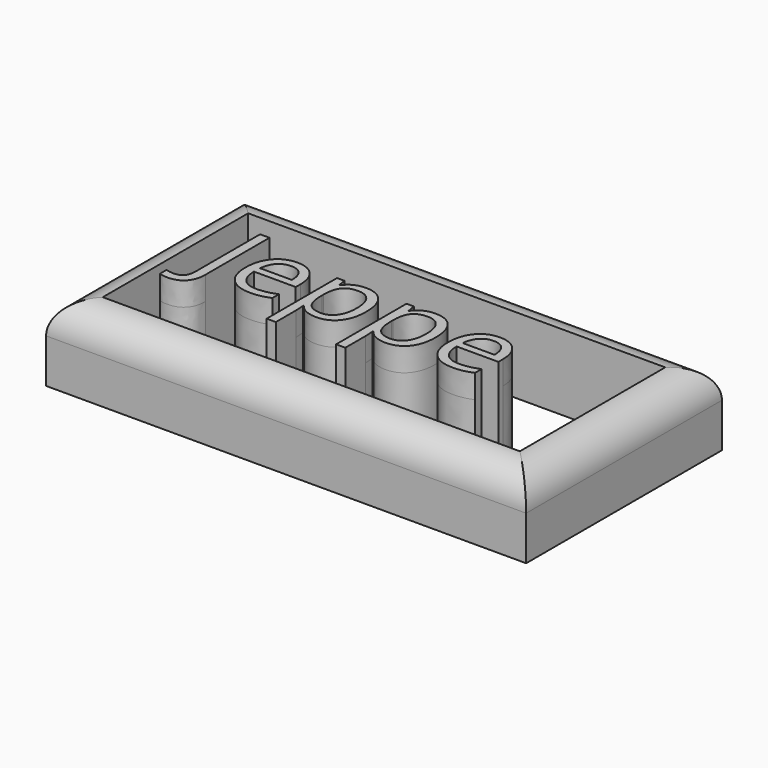
from build123d import *

# Parameters (mm, degrees)
F0_W         = 77.459409833
F0_H         = 39.4822433591
F1_DEPTH     = 12.192
F2_R         = 5.08
F3_TEXT_SIZE = 18.2969172278
F4_DEPTH     = 3.81
F6_DEPTH     = 25.4


# Not quite as in the source:
# - Text() gives the source's letters only with a copy of the font that has no kerning and outlines rounded to 1/6400 em; it was checked with that copy


with BuildPart() as f1:
    # F0 (on Top) → F1 (new body)
    with BuildSketch(Plane.XY):
        with Locations((4.5470893383, -5.5234562606)):
            Rectangle(F0_W, F0_H)
    extrude(amount=F1_DEPTH)

    # F2
    f2_edges = [f1.edges().sort_by_distance(p)[0] for p in [
        (4.547089, -25.264578, 12.192),
        (4.547089, 14.217665, 12.192),
        (43.276794, -5.523456, 12.192),
        (-34.182616, -5.523456, 12.192),
    ]]
    fillet(f2_edges, radius=F2_R)

    # F3 (on face) → F4 (join)
    with BuildSketch(Plane.XY.offset(12.192)):
        with Locations((-21.473845467, -13.173780404)):
            Text('Jeppe', F3_TEXT_SIZE, font='Open Sans', text_align=(TextAlign.LEFT, TextAlign.BOTTOM))
    extrude(amount=F4_DEPTH)

    # F6 (cut): a face of the model
    f6_faces = [f1.faces().sort_by_distance(p)[0] for p in [
        (4.9159619401, -5.0083097762, 12.192),
    ]]
    extrude(f6_faces, amount=-F6_DEPTH, mode=Mode.SUBTRACT)


solid = f1.part
